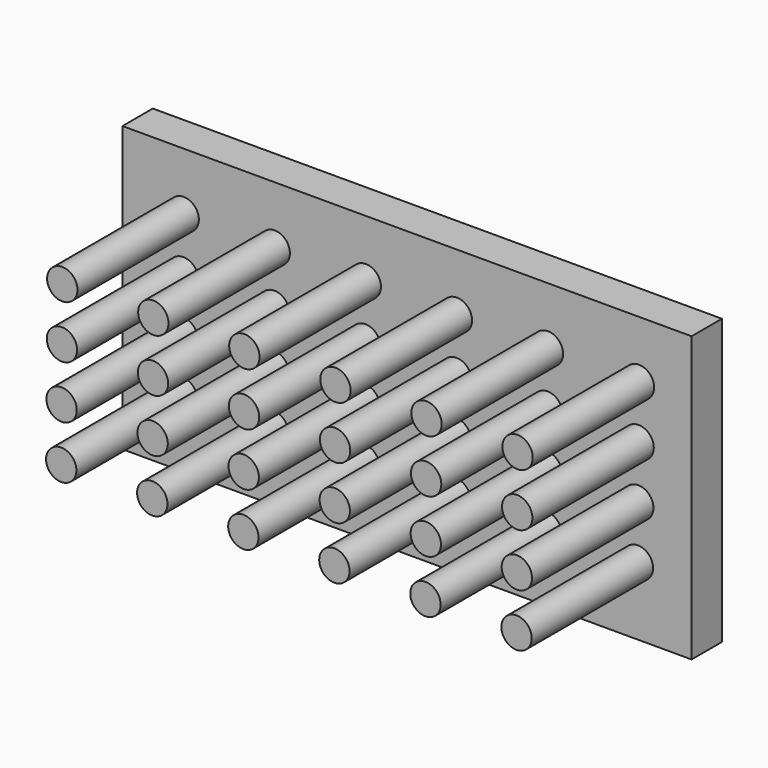
from build123d import *

# Parameters (mm, degrees)
F0_W     = 38.1
F0_H     = 19.05
F1_DEPTH = 2.54
F2_R     = 1.016
F3_DEPTH = 10.16
F4_DEPTH = 10.16


# Not quite as in the source:
# - a feature names something its author has since deleted; it is built from what else it names


with BuildPart() as f1:
    # F0 (on Front) → F1 (new body)
    with BuildSketch(Plane.XZ):
        Rectangle(F0_W, F0_H)
    extrude(amount=F1_DEPTH)

    # F2 (on face) → F3 (join)
    with BuildSketch(Plane.XZ.offset(2.54)):
        with Locations((-14.9520980194, 5.6684408337)):
            Circle(F2_R)
        with Locations((-8.8560991403, 5.6721375078)):
            Circle(F2_R)
        with Locations((-8.8793454933, 2.1162134919)):
            Circle(F2_R)
        with Locations((-14.9753443725, 2.1125168178)):
            Circle(F2_R)
        with Locations((-14.9985907255, -1.4434071982)):
            Circle(F2_R)
        with Locations((-8.9025918464, -1.439710524)):
            Circle(F2_R)
        with Locations((-8.9258381994, -4.99563454)):
            Circle(F2_R)
        with Locations((-15.0218370786, -4.9993312141)):
            Circle(F2_R)
        with Locations((-2.8298393203, -4.9919378658)):
            Circle(F2_R)
        with Locations((-2.8065929672, -1.4360138499)):
            Circle(F2_R)
        with Locations((-2.7833466142, 2.119910166)):
            Circle(F2_R)
        with Locations((-2.7601002611, 5.675834182)):
            Circle(F2_R)
        with Locations((3.335898618, 5.6795308561)):
            Circle(F2_R)
        with Locations((3.312652265, 2.1236068402)):
            Circle(F2_R)
        with Locations((3.2894059119, -1.4323171757)):
            Circle(F2_R)
        with Locations((3.2661595589, -4.9882411917)):
            Circle(F2_R)
    extrude(amount=F3_DEPTH)

    # F2 (on face) → F4 (join)
    with BuildSketch(Plane.XZ.offset(2.54)):
        with Locations((9.4318974972, 5.6832275303)):
            Circle(F2_R)
        with Locations((9.4086511441, 2.1273035143)):
            Circle(F2_R)
        with Locations((9.3854047911, -1.4286205016)):
            Circle(F2_R)
        with Locations((9.362158438, -4.9845445175)):
            Circle(F2_R)
        with Locations((15.4581573172, -4.9808478434)):
            Circle(F2_R)
        with Locations((15.4814036702, -1.4249238275)):
            Circle(F2_R)
        with Locations((15.5046500233, 2.1310001885)):
            Circle(F2_R)
        with Locations((15.5278963763, 5.6869242044)):
            Circle(F2_R)
    extrude(amount=F4_DEPTH)


solid = f1.part
